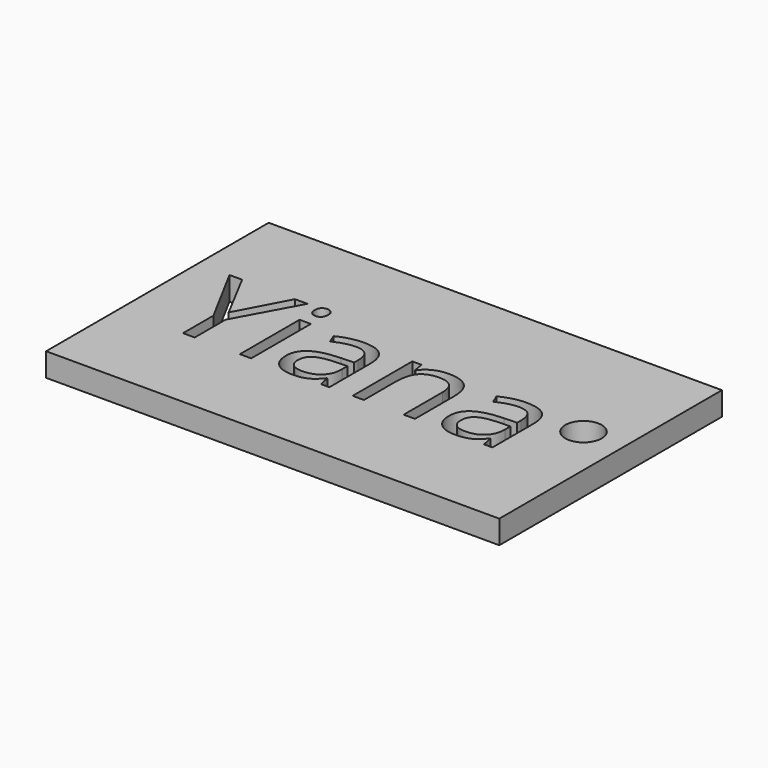
from build123d import *

# Parameters (mm, degrees)
F0_W         = 116.0313077271
F0_H         = 71.2362155318
F1_DEPTH     = 6
F2_R         = 4.658602171
F2_TEXT_SIZE = 35.6744704571
F3_DEPTH     = 6


# Not quite as in the source:
# - Text() gives the source's letters only with a copy of the font that has no kerning and outlines rounded to 1/6400 em; it was checked with that copy


with BuildPart() as f1:
    # F0 (on Top) → F1 (new body)
    with BuildSketch(Plane.XY):
        with Locations((-19.5326562971, 0.3007799387)):
            Rectangle(F0_W, F0_H)
    extrude(amount=F1_DEPTH)

    # F2 (on face) → F3 (cut)
    with BuildSketch(Plane.XY.offset(6)):
        with Locations((28.1079839915, 4.5887483284)):
            Circle(F2_R)
        with Locations((-69.5384087282, -12.1115120899)):
            Text('Yiana', F2_TEXT_SIZE, font='Open Sans', text_align=(TextAlign.LEFT, TextAlign.BOTTOM))
    extrude(amount=-F3_DEPTH, mode=Mode.SUBTRACT)


solid = f1.part
